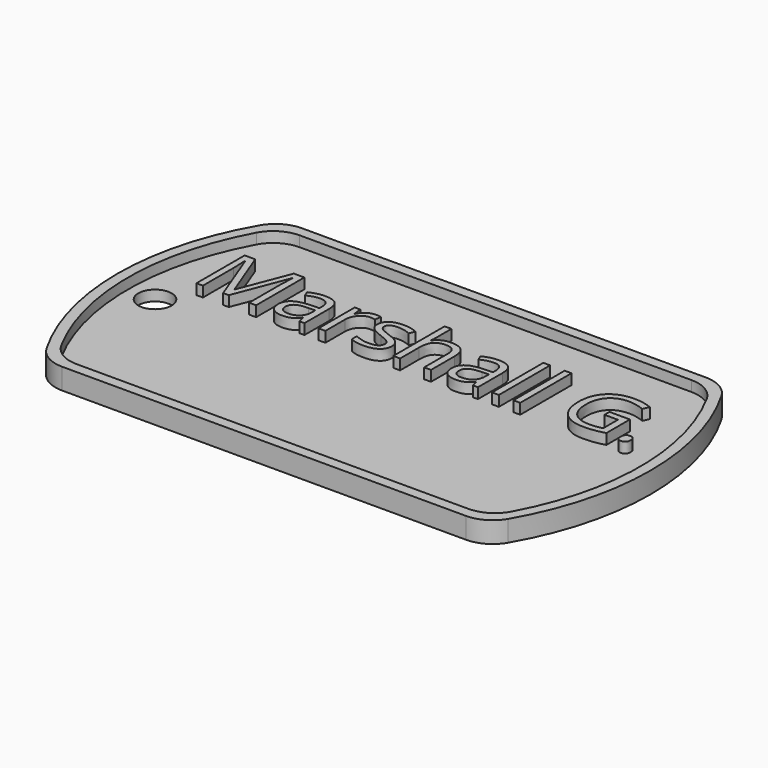
from build123d import *

# Parameters (mm, degrees)
F1_DEPTH     = 1
F3_DEPTH     = 1
F4_R         = 1.5875
F5_DEPTH     = 1
F6_TEXT_SIZE = 8.0429638426
F7_DEPTH     = 1


# Not quite as in the source:
# - Text() gives the source's letters only with a copy of the font that has no kerning and outlines rounded to 1/6400 em; it was checked with that copy


with BuildPart() as f1:
    # F0 (on Top) → F1 (new body)
    with BuildSketch(Plane.XY):
        with BuildLine():
            ThreePointArc((-19.2474145991, 14.2875), (-20.8349145991, 13.862130657), (-21.9970452561, 12.7))
            ThreePointArc((-21.9970452561, 12.7), (-25.4, 0), (-21.9970452561, -12.7))
            ThreePointArc((-21.9970452561, -12.7), (-20.8349145991, -13.862130657), (-19.2474145991, -14.2875))
            Line((-19.2474145991, -14.2875), (19.2474145991, -14.2875))
            ThreePointArc((19.2474145991, -14.2875), (20.8349145991, -13.862130657), (21.9970452561, -12.7))
            ThreePointArc((21.9970452561, -12.7), (25.4, 0), (21.9970452561, 12.7))
            ThreePointArc((21.9970452561, 12.7), (20.8349145991, 13.862130657), (19.2474145991, 14.2875))
            Line((19.2474145991, 14.2875), (-19.2474145991, 14.2875))
        make_face()
    extrude(amount=F1_DEPTH)

    # F2 (on face) → F3 (join)
    with BuildSketch(Plane.XY.offset(1)):
        with BuildLine():
            Line((19.2474145991, 14.2875), (-19.2474145991, 14.2875))
            ThreePointArc((-19.2474145991, 14.2875), (-20.8349145991, 13.862130657), (-21.9970452561, 12.7))
            ThreePointArc((-21.9970452561, 12.7), (-25.4, 0), (-21.9970452561, -12.7))
            ThreePointArc((-21.9970452561, -12.7), (-20.8349145991, -13.862130657), (-19.2474145991, -14.2875))
            Line((-19.2474145991, -14.2875), (19.2474145991, -14.2875))
            ThreePointArc((19.2474145991, -14.2875), (20.8349145991, -13.862130657), (21.9970452561, -12.7))
            ThreePointArc((21.9970452561, -12.7), (25.4, 0), (21.9970452561, 12.7))
            ThreePointArc((21.9970452561, 12.7), (20.8349145991, 13.862130657), (19.2474145991, 14.2875))
        make_face()
        with BuildLine():
            ThreePointArc((-21.4526124879, 11.6252061249), (-20.2856017842, 12.8404540819), (-18.6611352482, 13.2875))
            Line((-18.6611352482, 13.2875), (18.6611352482, 13.2875))
            ThreePointArc((18.6611352482, 13.2875), (20.2856017842, 12.8404540819), (21.4526124879, 11.6252061249))
            ThreePointArc((21.4526124879, 11.6252061249), (24.4, 0), (21.4526124879, -11.6252061249))
            ThreePointArc((21.4526124879, -11.6252061249), (20.2856017842, -12.8404540819), (18.6611352482, -13.2875))
            Line((18.6611352482, -13.2875), (-18.6611352482, -13.2875))
            ThreePointArc((-18.6611352482, -13.2875), (-20.2856017842, -12.8404540819), (-21.4526124879, -11.6252061249))
            ThreePointArc((-21.4526124879, -11.6252061249), (-24.4, 0), (-21.4526124879, 11.6252061249))
        make_face(mode=Mode.SUBTRACT)
    extrude(amount=F3_DEPTH)

    # F4 (on face) → F5 (cut)
    with BuildSketch(Plane.XY.offset(1)):
        with Locations((-21.821282804, 0)):
            Circle(F4_R)
    extrude(amount=-F5_DEPTH, mode=Mode.SUBTRACT)

    # F6 (on face) → F7 (join)
    with BuildSketch(Plane.XY.offset(1)):
        with Locations((-20.6310991198, 2.4615060538)):
            Text('Marshall G.', F6_TEXT_SIZE, font='Open Sans', text_align=(TextAlign.LEFT, TextAlign.BOTTOM))
    extrude(amount=F7_DEPTH)


solid = f1.part
